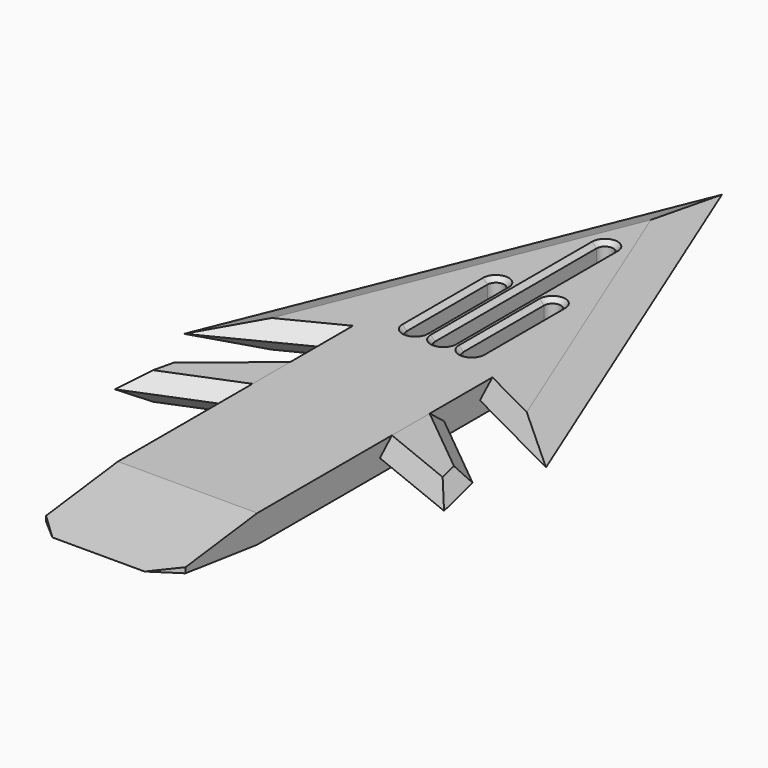
from build123d import *

# Parameters (mm, degrees)
F1_DEPTH   = 6.35
F2_DEPTH   = 6.35
F3_DEPTH   = 6.35
F4_SIZE2   = 3.175
F4_SIZE    = 7.62
F4_2_SIZE2 = 3.17499
F4_2_SIZE  = 7.61999
F5_SIZE2   = 3.17499
F5_SIZE    = 3.17499
F6_SIZE2   = 3.17499
F6_SIZE    = 3.17499
F6_2_SIZE2 = 3.17499
F6_2_SIZE  = 3.17499
F7_SIZE    = 1.016
F8_SIZE2   = 3.175
F8_SIZE    = 25.4
F8_2_SIZE2 = 3.17499
F8_2_SIZE  = 25.39999


# Not quite as in the source:
# - a fillet or chamfer is up to 0.001 mm smaller than in the source, because OpenCascade refuses the exact size


with BuildPart() as f1:
    # F0 (on Top) → F1 (new body)
    with BuildSketch(Plane.XY):
        Polygon((41.275, -12.8728821874), (0, 88.9), (-41.275, -12.8728821874), (-15.9091800451, 0), (-15.9091800451, -10.2451825514), (-15.9091800451, -28.5296985704), (-15.9091800451, -83.9729532599), (-10.527680628, -88.9), (10.527680628, -88.9), (15.9091800451, -83.9729532599), (15.9091800451, -28.5296985704), (15.9091800451, -10.2451825514), (15.9091800451, 0), align=None)
        with BuildLine():
            Line((-8.355671237, 9.4862803817), (-8.355671237, 32.5063206255))
            ThreePointArc((-8.355671237, 32.5063206255), (-6.450671237, 34.4113206255), (-4.545671237, 32.5063206255))
            Line((-4.545671237, 32.5063206255), (-4.545671237, 9.4862803817))
            ThreePointArc((-4.545671237, 9.4862803817), (-6.450671237, 7.5812803817), (-8.355671237, 9.4862803817))
        make_face(mode=Mode.SUBTRACT)
        with BuildLine():
            Line((4.545671237, 9.4862803817), (4.545671237, 32.5063206255))
            ThreePointArc((4.545671237, 32.5063206255), (6.450671237, 34.4113206255), (8.355671237, 32.5063206255))
            Line((8.355671237, 32.5063206255), (8.355671237, 9.4862803817))
            ThreePointArc((8.355671237, 9.4862803817), (6.450671237, 7.5812803817), (4.545671237, 9.4862803817))
        make_face(mode=Mode.SUBTRACT)
        with BuildLine():
            Line((-1.905, 9.4862803817), (-1.905, 55.5263608694))
            ThreePointArc((-1.905, 55.5263608694), (0, 57.4313608694), (1.905, 55.5263608694))
            Line((1.905, 55.5263608694), (1.905, 9.4862803817))
            ThreePointArc((1.905, 9.4862803817), (0, 7.5812803817), (-1.905, 9.4862803817))
        make_face(mode=Mode.SUBTRACT)
    extrude(amount=F1_DEPTH)

    # F4
    f4_edges = [f1.edges().sort_by_distance(p)[0] for p in [
        (-20.6375, 38.013559, 0),
        (20.6375, 38.013559, 0),
    ]]
    f4_side = f1.faces().sort_by_distance((0, -6.764351, 0))[0]
    chamfer(f4_edges, length=F4_SIZE, length2=F4_SIZE2, reference=f4_side)

    # F4#2 (size 7.62 and 3.175 in the source; OpenCascade refuses exactly that, so slightly less here)
    f4_2_edges = [f1.edges().sort_by_distance(p)[0] for p in [
        (20.6375, 38.013559, 6.35),
        (-20.6375, 38.013559, 6.35),
    ]]
    f4_2_side = f1.faces().sort_by_distance((0, -6.764351, 6.35))[0]
    chamfer(f4_2_edges, length=F4_2_SIZE, length2=F4_2_SIZE2, reference=f4_2_side)

    # F5 (size 3.175 and 3.175 in the source; OpenCascade refuses exactly that, so slightly less here)
    f5_edges = [f1.edges().sort_by_distance(p)[0] for p in [
        (23.41519, -3.80922, 6.35),
        (23.415183, -3.809216, 0),
        (-23.41519, -3.80922, 6.35),
        (-23.415183, -3.809216, 0),
    ]]
    chamfer(f5_edges, length=F5_SIZE, length2=F5_SIZE2)

    # F7
    f7_edges = [f1.edges().sort_by_distance(p)[0] for p in [
        (-8.355671, 20.996301, 6.35),
        (-6.450671, 7.58128, 6.35),
        (-4.545671, 20.996301, 6.35),
        (-6.450671, 34.411321, 6.35),
        (-1.905, 32.506321, 6.35),
        (0, 7.58128, 6.35),
        (1.905, 32.506321, 6.35),
        (0, 57.431361, 6.35),
        (8.355671, 20.996301, 6.35),
        (6.450671, 34.411321, 6.35),
        (4.545671, 20.996301, 6.35),
        (6.450671, 7.58128, 6.35),
        (-6.450671, 7.58128, 0),
        (0, 7.58128, 0),
        (6.450671, 7.58128, 0),
        (4.545671, 20.996301, 0),
        (8.355671, 20.996301, 0),
        (-1.905, 32.506321, 0),
        (1.905, 32.506321, 0),
        (-4.545671, 20.996301, 0),
        (-8.355671, 20.996301, 0),
        (6.450671, 34.411321, 0),
        (-6.450671, 34.411321, 0),
        (0, 57.431361, 0),
    ]]
    chamfer(f7_edges, length=F7_SIZE)

    # F8
    f8_edges = [f1.edges().sort_by_distance(p)[0] for p in [
        (0, -88.9, 6.35),
    ]]
    f8_side = f1.faces().sort_by_distance((0, -23.545695, 6.35))[0]
    chamfer(f8_edges, length=F8_SIZE, length2=F8_SIZE2, reference=f8_side)

    # F8#2 (size 25.4 and 3.175 in the source; OpenCascade refuses exactly that, so slightly less here)
    f8_2_edges = [f1.edges().sort_by_distance(p)[0] for p in [
        (0, -88.9, 0),
    ]]
    f8_2_side = f1.faces().sort_by_distance((0, -23.545717, 0))[0]
    chamfer(f8_2_edges, length=F8_2_SIZE, length2=F8_2_SIZE2, reference=f8_2_side)


with BuildPart() as f2:
    # F0 (on Top) → F2 (new body)
    with BuildSketch(Plane.XY):
        Polygon((-15.9091800451, -28.5296985704), (-15.9091800451, -10.2451825514), (-34.7830280662, -25.6761983037), (-37.5656671822, -37.3127013445), align=None)
    extrude(amount=F2_DEPTH)

    # F6 (size 3.175 and 3.175 in the source; OpenCascade refuses exactly that, so slightly less here)
    f6_edges = [f2.edges().sort_by_distance(p)[0] for p in [
        (-25.346104, -17.96069, 6.35),
        (-25.346104, -17.96069, 0),
        (-36.174348, -31.49445, 6.35),
        (-36.174348, -31.49445, 0),
        (-26.737424, -32.9212, 0),
        (-26.737424, -32.9212, 6.35),
    ]]
    chamfer(f6_edges, length=F6_SIZE, length2=F6_SIZE2)


with BuildPart() as f3:
    # F0 (on Top) → F3 (new body)
    with BuildSketch(Plane.XY):
        Polygon((34.7830280662, -25.6761983037), (15.9091800451, -10.2451825514), (15.9091800451, -28.5296985704), (37.5656671822, -37.3127013445), align=None)
    extrude(amount=F3_DEPTH)

    # F6#2 (size 3.175 and 3.175 in the source; OpenCascade refuses exactly that, so slightly less here)
    f6_2_edges = [f3.edges().sort_by_distance(p)[0] for p in [
        (25.346104, -17.96069, 6.35),
        (25.346104, -17.96069, 0),
        (36.174348, -31.49445, 0),
        (36.174348, -31.49445, 6.35),
        (26.737424, -32.9212, 6.35),
        (26.737424, -32.9212, 0),
    ]]
    chamfer(f6_2_edges, length=F6_2_SIZE, length2=F6_2_SIZE2)


solid = Compound([f1.part, f2.part, f3.part])
